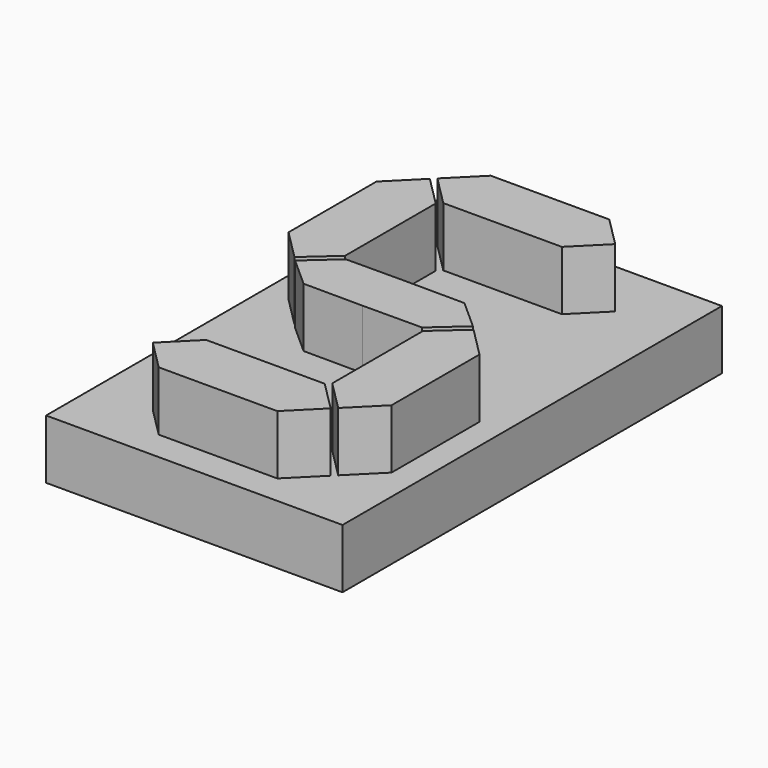
from build123d import *

# Parameters (mm, degrees)
F0_W     = 10
F0_H     = 16
F1_DEPTH = 2
F3_DEPTH = 2


# Not quite as in the source:
# - ends of sketch curves that miss each other by under 0.0002 mm in the source are joined


with BuildPart() as f1:
    # F0 (on Top) → F1 (new body)
    with BuildSketch(Plane.XY):
        Rectangle(F0_W, F0_H)
    extrude(amount=F1_DEPTH)

    # F2 (on face) → F3 (join)
    with BuildSketch(Plane.XY.offset(2)):
        Polygon((0, 7), (-2, 7), (-3, 6), (-2, 5), (0, 5), (2, 5), (3, 6), (2, 7), align=None)
        Polygon((-2.1414213562, 4.8585786438), (-3.1414213562, 5.8585786438), (-4.1414213562, 4.8585786438), (-4.1414213562, 1.1507223826), (-3.1374518146, 0.1453992321), (-2.1414213562, 1.0335195075), align=None)
        Polygon((2, 0.891659756), (2.00782e-05, 0.9006214721), (-2, 0.891659756), (-3, 0), (-2, -0.891659756), (-2.00782e-05, -0.9006214721), (2, -0.891659756), (3, 0), align=None)
        Polygon((0, -5), (-2, -5), (-3, -6), (-2, -7), (0, -7), (2, -7), (3, -6), (2, -5), align=None)
        Polygon((3.1374518146, -0.1453992321), (2.1414213562, -1.0335195075), (2.1414213562, -4.8585786438), (3.1414213562, -5.8585786438), (4.1414213562, -4.8585786438), (4.1414213562, -1.1507223826), align=None)
    extrude(amount=F3_DEPTH)


solid = f1.part
